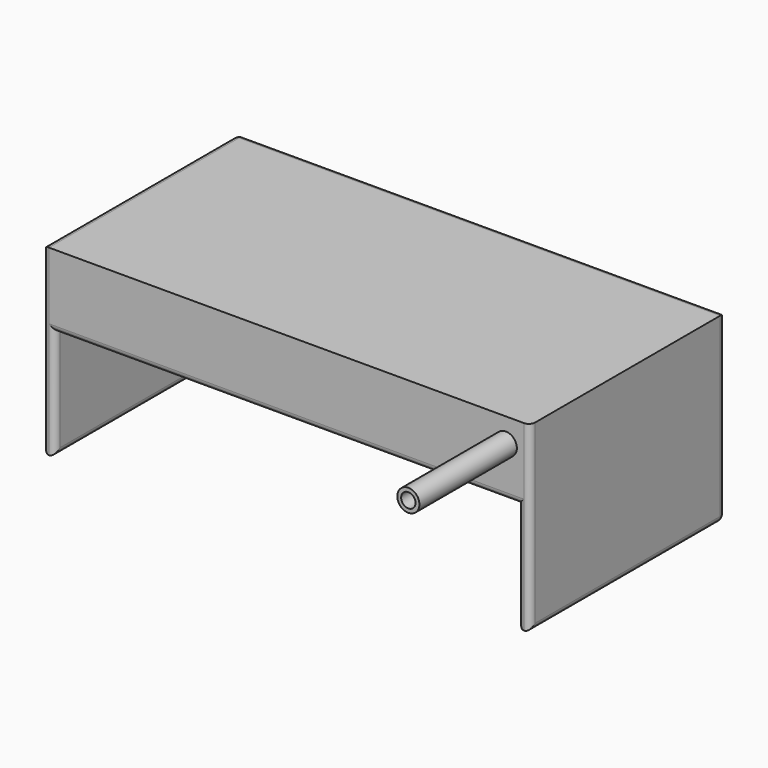
from build123d import *

# Parameters (mm, degrees)
F0_W      = 4000
F0_H      = 2000
F1_DEPTH  = 1500
F2_W      = 3800
F2_H      = 900
F3_DEPTH  = 1900
F4_W      = 3800
F4_H      = 1800
F5_DEPTH  = 500
F6_R      = 90.7224543957
F6_R_2    = 58.9600889745
F7_DEPTH  = 1000
F8_R      = 49.99999
F9_R      = 58.4664374667
F10_DEPTH = 100


# Not quite as in the source:
# - a fillet or chamfer is up to 0.001 mm smaller than in the source, because OpenCascade refuses the exact size


with BuildPart() as f1:
    # F0 (on Top) → F1 (new body)
    with BuildSketch(Plane.XY):
        with Locations((20.9405645728, -183.9094895178)):
            Rectangle(F0_W, F0_H)
    extrude(amount=F1_DEPTH)

    # F2 (on face) → F3 (cut)
    with BuildSketch(Plane.XZ.offset(1183.9094895178)):
        with Locations((20.9405645728, 450)):
            Rectangle(F2_W, F2_H)
    extrude(amount=-F3_DEPTH, mode=Mode.SUBTRACT)

    # F4 (on face) → F5 (cut)
    with BuildSketch(Plane(origin=(0, 0, 900), x_dir=(1, 0, 0), z_dir=(0, 0, -1))):
        with Locations((20.9405645728, 183.9094895178)):
            Rectangle(F4_W, F4_H)
    extrude(amount=-F5_DEPTH, mode=Mode.SUBTRACT)

    # F6 (on face) → F7 (join)
    with BuildSketch(Plane.XZ.offset(1183.9094895178)):
        with Locations((1820.9405645728, 1300)):
            Circle(F6_R)
        with Locations((1820.9405645728, 1300)):
            Circle(F6_R_2, mode=Mode.SUBTRACT)
    extrude(amount=F7_DEPTH)

    # F8 (radius 50 in the source; OpenCascade refuses exactly that, so slightly less here)
    f8_edges = [f1.edges().sort_by_distance(p)[0] for p in [
        (20.940565, -1183.90949, 900),
        (-1979.059435, -1183.90949, 750),
        (2020.940565, -1183.90949, 750),
        (2020.940565, 816.09051, 750),
        (-1979.059435, 816.09051, 750),
        (20.940565, -1083.90949, 900),
        (20.940565, 816.09051, 0),
        (-1979.059435, -183.90949, 0),
        (-1979.059435, -183.90949, 1500),
        (-1879.059435, -233.90949, 0),
        (1920.940565, -233.90949, 0),
        (2020.940565, -183.90949, 0),
        (1920.940565, -1183.90949, 450),
        (-1879.059435, -1183.90949, 450),
        (20.940565, 716.09051, 1400),
        (-1879.059435, -183.90949, 1400),
        (1920.940565, -183.90949, 1400),
        (20.940565, -1083.90949, 1400),
        (20.940565, 816.09051, 1500),
        (1920.940565, 716.09051, 700),
        (-1879.059435, 716.09051, 700),
        (20.940565, 716.09051, 0),
    ]]
    fillet(f8_edges, radius=F8_R)

    # F9 (on face) → F10 (cut)
    with BuildSketch(Plane.XZ.offset(1183.9094895178)):
        with Locations((1820.9405645728, 1300)):
            Circle(F9_R)
    extrude(amount=-F10_DEPTH, mode=Mode.SUBTRACT)


solid = f1.part
